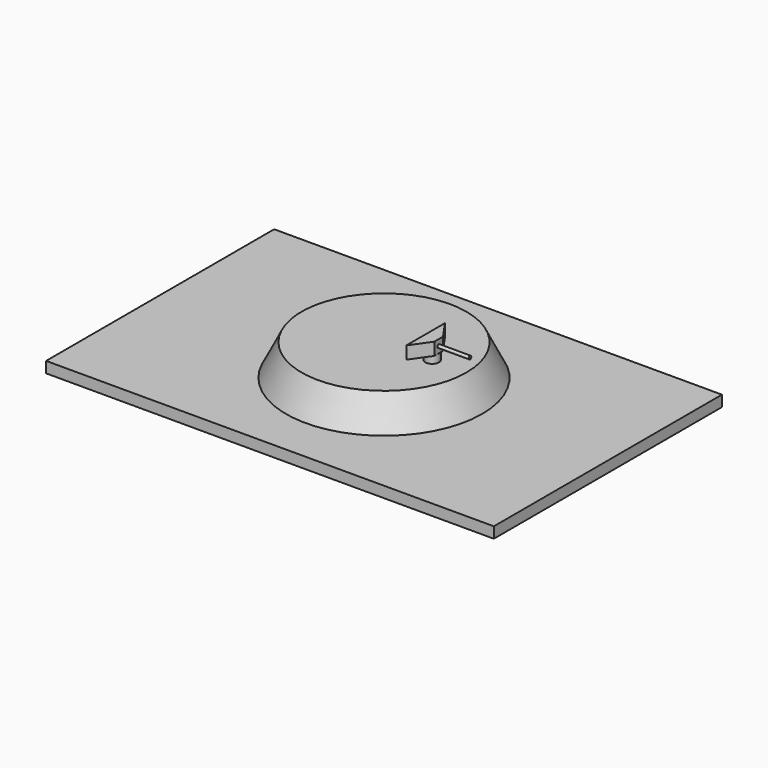
from build123d import *

# Parameters (mm, degrees)
F0_W         = 72.464676
F0_H         = 46.138592
F1_DEPTH     = 1.778
F2_R         = 15.875
F4_R         = 13.341257797
F6_R         = 1.1014910557
F7_DEPTH     = 1.27
F9_DEPTH     = 2.032
F10_T1_DEPTH = 15.1513653298
F11_R        = 0.2563999908
F12_DEPTH    = 5.08


# Not quite as in the source:
# - a fillet or chamfer that OpenCascade refuses, or shapes differently, is made with other operations: its cross-section is extruded or revolved along the edge and cut away or added


with BuildPart() as f1:
    # F0 (on Top) → F1 (new body)
    with BuildSketch(Plane.XY):
        Rectangle(F0_W, F0_H)
    extrude(amount=F1_DEPTH)

    # F2 (on face) → F5 section 0
    with BuildSketch(Plane.XY.offset(1.778)):
        Circle(F2_R)
    # F4 (on offset) → F5 section 1
    with BuildSketch(Plane.XY.offset(6.858)):
        Circle(F4_R)
    loft()

    # F6 (on face) → F7 (join)
    with BuildSketch(Plane.XY.offset(6.858)):
        with Locations((7.7888662927, 0)):
            Circle(F6_R)
    extrude(amount=F7_DEPTH)

    # F8 (on face) → F9 (join)
    with BuildSketch(Plane.XY.offset(8.128)):
        with BuildLine():
            Line((6.7317243665, -0.3094082962), (6.7317243665, -5.9662871063))
            Line((6.7317243665, -5.9662871063), (8.8460082188, -5.9662871063))
            Line((8.8460082188, -5.9662871063), (8.8460082188, -0.3094082962))
            ThreePointArc((8.8460082188, -0.3094082962), (7.7888662927, -1.1014910557), (6.7317243665, -0.3094082962))
        make_face()
        with BuildLine():
            Line((6.7317243665, 5.9662871063), (6.7317243665, 0.3094082962))
            ThreePointArc((6.7317243665, 0.3094082962), (7.7888662927, 1.1014910557), (8.8460082188, 0.3094082962))
            Line((8.8460082188, 0.3094082962), (8.8460082188, 5.9662871063))
            Line((8.8460082188, 5.9662871063), (6.7317243665, 5.9662871063))
        make_face()
        with BuildLine():
            Line((6.7317243665, 0.3094082962), (6.7317243665, -0.3094082962))
            ThreePointArc((6.7317243665, -0.3094082962), (7.7888662927, -1.1014910557), (8.8460082188, -0.3094082962))
            Line((8.8460082188, -0.3094082962), (8.8460082188, 0.3094082962))
            ThreePointArc((8.8460082188, 0.3094082962), (7.7888662927, 1.1014910557), (6.7317243665, 0.3094082962))
        make_face()
    extrude(amount=F9_DEPTH)

    # F10: chamfer of 5.08 x 3.5570542941 on 2 edges, made by hand

    # F10_s2 → F10_t1 (cut)
    with BuildSketch(Plane.XY.offset(8.128)):
        Polygon((8.8460082188, -0.8862871063), (5.2889539247, -5.9662871063), (8.8460082188, -5.9662871063), align=None)
        Polygon((8.8460082188, 0.8862871063), (5.2889539247, 5.9662871063), (8.8460082188, 5.9662871063), align=None)
    extrude(amount=F10_T1_DEPTH, mode=Mode.SUBTRACT)

    # F11 (on face) → F12 (join)
    with BuildSketch(Plane.YZ.offset(8.8460082188)):
        with Locations((0, 9.1775208712)):
            Circle(F11_R)
    extrude(amount=F12_DEPTH)


solid = f1.part
